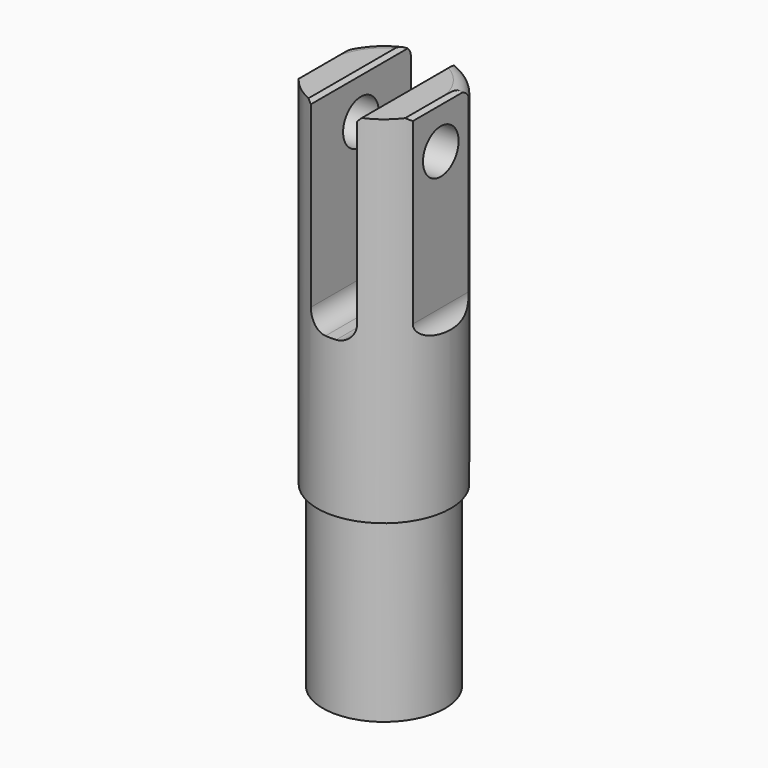
from build123d import *

# Parameters (mm, degrees)
F0_R           = 8.7249
F1_DEPTH       = 25.4
F2_R           = 9.525
F3_DEPTH       = 50.8
F4_W           = 6.604
F4_H           = 31.75
F4_W_2         = 7.7840778498
F4_H_2         = 37.4901928008
F5_DEPTH       = 25.4
F5_DEPTH_BACK  = 25.4
F6_R           = 2.54
F7_SIZE        = 0.508
F8_T4_DEPTH    = 22.6820176921
F8_S5_R        = 9.525
F8_T6_DEPTH    = 13
F8_T10_DEPTH   = 22.6820176921
F8_S11_R       = 9.525
F8_T12_DEPTH   = 13
F9_R           = 3.175
F10_DEPTH      = 25.4
F10_DEPTH_BACK = 25.4
F11_R          = 1.778
F12_R          = 6.35
F13_DEPTH      = 25.4


# Not quite as in the source:
# - a fillet or chamfer that OpenCascade refuses, or shapes differently, is made with other operations: its cross-section is extruded or revolved along the edge and cut away or added


with BuildPart() as f1:
    # F0 (on Top) → F1 (new body)
    with BuildSketch(Plane.XY):
        Circle(F0_R)
    extrude(amount=F1_DEPTH)

    # F2 (on face) → F3 (join)
    with BuildSketch(Plane.XY.offset(25.4)):
        Circle(F2_R)
    extrude(amount=F3_DEPTH)

    # F4 (on Front) → F5 (cut, two sides)
    with BuildSketch(Plane.XZ) as f5_sk:
        with Locations((0, 63.5)):
            Rectangle(F4_W, F4_H)
        with Locations((12.0047114623, 66.3700964004)):
            Rectangle(F4_W_2, F4_H_2)
        with Locations((-12.0047114623, 66.3700964004)):
            Rectangle(F4_W_2, F4_H_2)
    extrude(amount=-F5_DEPTH, mode=Mode.SUBTRACT)
    extrude(f5_sk.sketch, amount=F5_DEPTH_BACK, mode=Mode.SUBTRACT)

    # F6
    f6_edges = [f1.edges().sort_by_distance(p)[0] for p in [
        (-3.302, 0, 47.625),
        (3.302, 0, 47.625),
    ]]
    fillet(f6_edges, radius=F6_R)

    # F7
    f7_edges = [f1.edges().sort_by_distance(p)[0] for p in [
        (3.302, 0, 76.2),
        (-3.302, 0, 76.2),
        (-8.112673, 0, 76.2),
        (8.112673, 0, 76.2),
    ]]
    chamfer(f7_edges, length=F7_SIZE)

    # F8: fillet of radius 2.54 on 2 edges, made by hand


with BuildPart() as f8_tool2:
    # F8_s3 → F8_t4 (new body)
    with BuildSketch(Plane.XZ.offset(11.341008846)):
        with BuildLine():
            ThreePointArc((8.1126725374, 50.165), (8.8566213132, 48.3689487758), (10.6526725374, 47.625))
            Line((10.6526725374, 47.625), (8.1126725374, 47.625))
            Line((8.1126725374, 47.625), (8.1126725374, 50.165))
        make_face()
    extrude(amount=-F8_T4_DEPTH)

    # F8_s5 → F8_t6 (intersect, symmetric)
    with BuildSketch(Plane.XY.offset(48.9)):
        Circle(F8_S5_R)
    extrude(amount=F8_T6_DEPTH, both=True, mode=Mode.INTERSECT)


with BuildPart() as f1_1:
    add(f1.part)

    # F8_t1: union F8_tool2
    add(f8_tool2.part)


with BuildPart() as f8_tool8:
    # F8_s9 → F8_t10 (new body)
    with BuildSketch(Plane.XZ.offset(11.341008846)):
        with BuildLine():
            ThreePointArc((-8.1126725374, 50.165), (-8.8566213132, 48.3689487758), (-10.6526725374, 47.625))
            Line((-10.6526725374, 47.625), (-8.1126725374, 47.625))
            Line((-8.1126725374, 47.625), (-8.1126725374, 50.165))
        make_face()
    extrude(amount=-F8_T10_DEPTH)

    # F8_s11 → F8_t12 (intersect, symmetric)
    with BuildSketch(Plane.XY.offset(48.9)):
        Circle(F8_S11_R)
    extrude(amount=F8_T12_DEPTH, both=True, mode=Mode.INTERSECT)


with BuildPart() as f1_2:
    add(f1_1.part)

    # F8_t7: union F8_tool8
    add(f8_tool8.part)

    # F9 (on face) → F10 (cut, two sides)
    with BuildSketch(Plane(origin=(-8.1126725374, 0, 0), x_dir=(0, -1, 0), z_dir=(-1, 0, 0))) as f10_sk:
        with Locations((0, 69.85)):
            Circle(F9_R)
    extrude(amount=-F10_DEPTH, mode=Mode.SUBTRACT)
    extrude(f10_sk.sketch, amount=F10_DEPTH_BACK, mode=Mode.SUBTRACT)

    # F11
    f11_edges = [f1_2.edges().sort_by_distance(p)[0] for p in [
        (-5.900452, 7.477318, 76.2),
        (5.900452, 7.477318, 76.2),
    ]]
    fillet(f11_edges, radius=F11_R)

    # F12 (on face) → F13 (cut)
    with BuildSketch(Plane(origin=(0, 0, 0), x_dir=(1, 0, 0), z_dir=(0, 0, -1))):
        Circle(F12_R)
    extrude(amount=-F13_DEPTH, mode=Mode.SUBTRACT)


solid = f1_2.part
